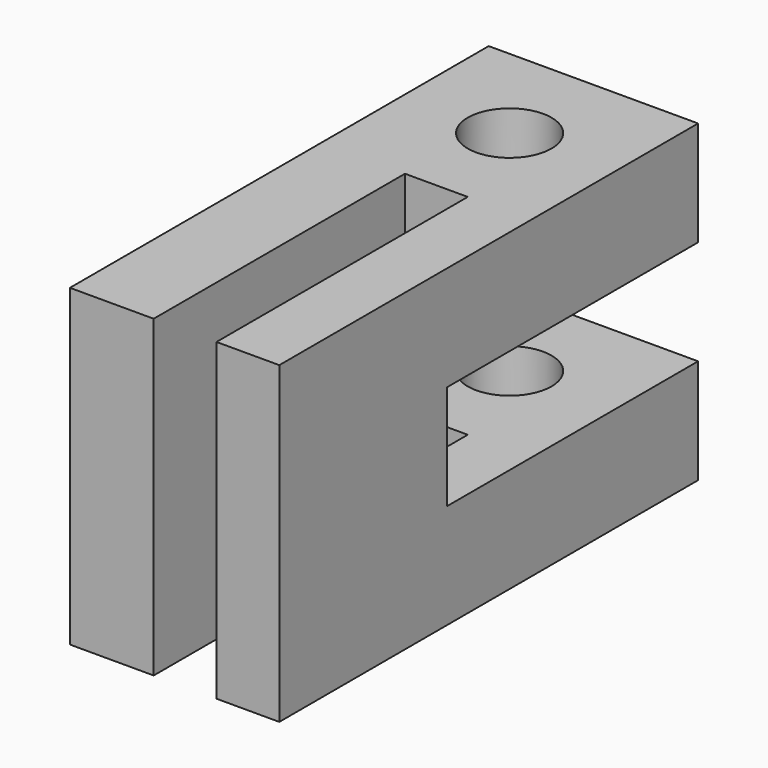
from build123d import *

# Parameters (mm, degrees)
F0_R     = 2
F1_DEPTH = 15
F2_W     = 15
F2_H     = 5
F3_DEPTH = 25.4


# Not quite as in the source:
# - a feature names something its author has since deleted; it is built from what else it names


with BuildPart() as f1:
    # F0 (on Top) → F1 (new body)
    with BuildSketch(Plane.XY):
        Polygon((-4, 0), (0, 0), (0, 15), (3, 15), (3, 0), (6, 0), (6, 25), (-4, 25), align=None)
        with Locations((1, 20)):
            Circle(F0_R, mode=Mode.SUBTRACT)
    extrude(amount=F1_DEPTH)

    # F2 (on face) → F3 (cut)
    with BuildSketch(Plane.YZ.offset(6)):
        with Locations((17.5, 7.5)):
            Rectangle(F2_W, F2_H)
    extrude(amount=-F3_DEPTH, mode=Mode.SUBTRACT)


solid = f1.part
